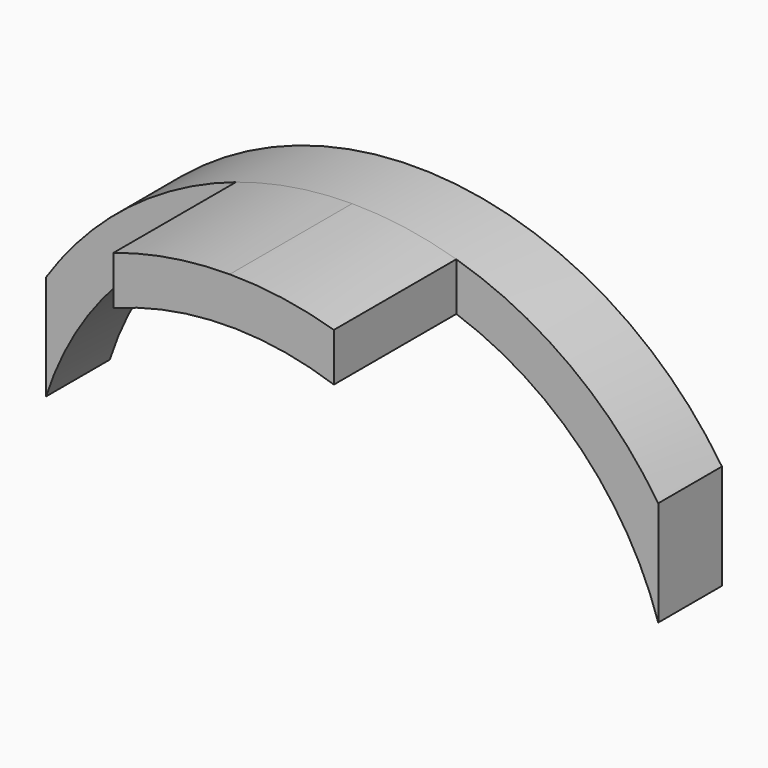
from build123d import *

# Parameters (mm, degrees)
F1_DEPTH = 3.302
F3_DEPTH = 6.35


with BuildPart() as f1:
    # F0 (on Front) → F1 (new body)
    with BuildSketch(Plane.XZ):
        with BuildLine():
            Line((12.7, 4.0659838908), (12.7, 8.4242269675))
            ThreePointArc((12.7, 8.4242269675), (0, 15.24), (-12.7, 8.4242269675))
            Line((-12.7, 8.4242269675), (-12.7, 4.0659838908))
            ThreePointArc((-12.7, 4.0659838908), (0, 13.335), (12.7, 4.0659838908))
        make_face()
    extrude(amount=F1_DEPTH)

    # F2 (on face) → F3 (join)
    with BuildSketch(Plane.XZ.offset(3.302)):
        with BuildLine():
            ThreePointArc((4.3219749297, 14.6143125978), (2.1835150571, 15.0827670537), (0, 15.24))
            ThreePointArc((0, 15.24), (-2.4425893067, 15.0429836628), (-4.8220250703, 14.4570285405))
            Line((-4.8220250703, 14.4570285405), (-4.8220250703, 12.4326304225))
            ThreePointArc((-4.8220250703, 12.4326304225), (-0.2661645943, 13.3323434327), (4.3219749297, 12.6151796542))
            Line((4.3219749297, 12.6151796542), (4.3219749297, 14.6143125978))
        make_face()
    extrude(amount=F3_DEPTH)


solid = f1.part
